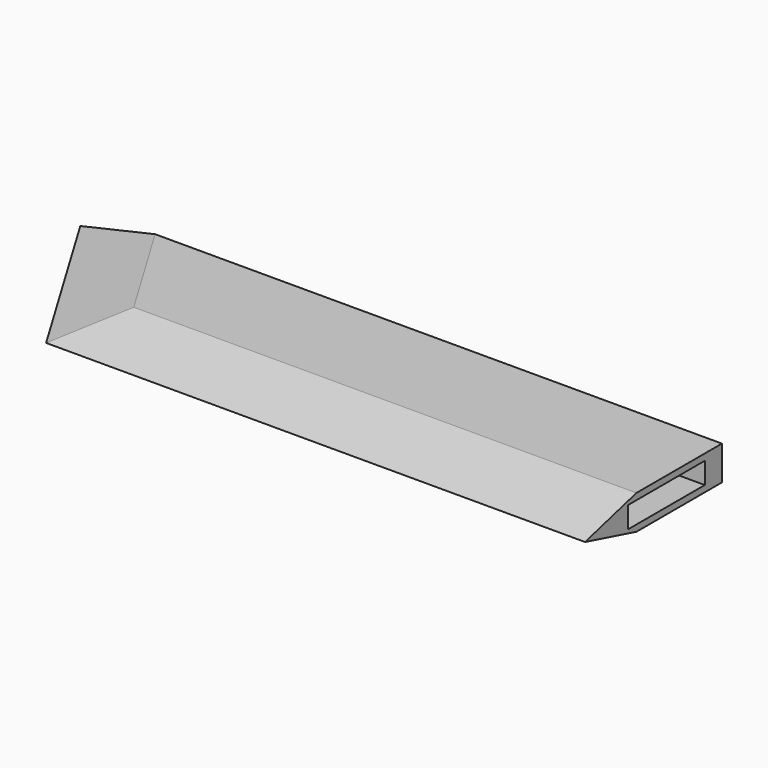
from build123d import *

# Parameters (mm, degrees)
F1_DEPTH = 8
F2_SIZE2 = 14.99999
F2_SIZE  = 3.99999
F3_SIZE2 = 4
F3_SIZE  = 15
F5_DEPTH = 50


# Not quite as in the source:
# - a fillet or chamfer is up to 0.001 mm smaller than in the source, because OpenCascade refuses the exact size


with BuildPart() as f1:
    # F0 (on Top) → F1 (new body)
    with BuildSketch(Plane.XY):
        Polygon((-126, 0), (0, 0), (0, 40), (-150, 40), align=None)
    extrude(amount=F1_DEPTH)

    # F2 (size 4 and 15 in the source; OpenCascade refuses exactly that, so slightly less here)
    f2_edges = [f1.edges().sort_by_distance(p)[0] for p in [
        (-63, 0, 8),
        (-138, 20, 8),
        (-63, 0, 0),
    ]]
    chamfer(f2_edges, length=F2_SIZE, length2=F2_SIZE2)

    # F3
    f3_edges = [f1.edges().sort_by_distance(p)[0] for p in [
        (-142.499997, 27.499995, 0),
    ]]
    f3_side = f1.faces().sort_by_distance((-71.315788, 27.719293, 0))[0]
    chamfer(f3_edges, length=F3_SIZE, length2=F3_SIZE2, reference=f3_side)

    # F4 (on face) → F5 (cut)
    with BuildSketch(Plane.YZ):
        Polygon((12.5, 6.5), (12.5, 4), (12.5, 1.5), (35, 1.5), (35, 6.5), align=None)
    extrude(amount=-F5_DEPTH, mode=Mode.SUBTRACT)


solid = f1.part
